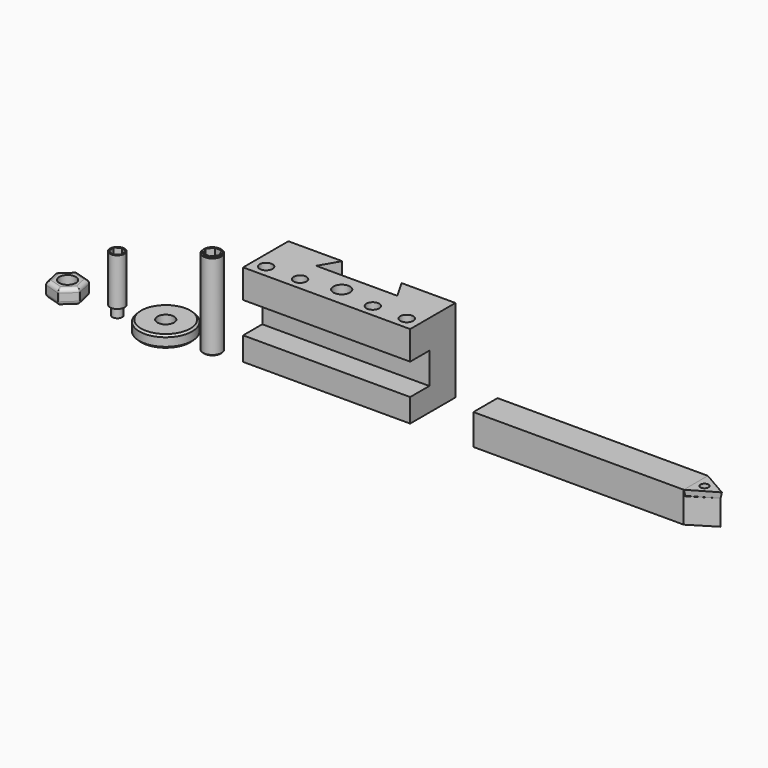
from build123d import *

# Parameters (mm, degrees)
F0_W      = 88.56
F0_H      = 12.4
F0_H_2    = 16.5
F0_H_3    = 15.22
F1_DEPTH  = 30
F2_DEPTH  = 12.7
F4_DEPTH  = 44.12
F5_D      = 6.8
F5_DEPTH  = 15.75
F5_TIP    = 2.0429261047
F6_D      = 8.8
F6_DEPTH  = 12
F6_TIP    = 2.6437867237
F7_R      = 4.9
F8_DEPTH  = 46
F9_SIZE   = 0.5
F11_DEPTH = 5
F12_R     = 14
F13_DEPTH = 6.43
F14_SIZE  = 1
F15_D     = 8.8
F16_R     = 2.6
F17_DEPTH = 5
F18_R     = 3.85
F19_DEPTH = 25
F21_DEPTH = 6.4
F23_DEPTH = 8
F24_D     = 8.8
F25_R     = 2
F26_R     = 0.5
F28_DEPTH = 16
F30_DEPTH = 13.3073726019
F32_DEPTH = 3
F32_TAPER = 7
F33_D     = 4.2
F33_DEPTH = 3
F33_TIP   = 1.2618073
F35_D     = 3.3


# Not quite as in the source:
# - a feature of the source that left no trace in its solid (it failed there, or was rolled back) is left out


with BuildPart() as f1:
    # F0 (on Front) → F1 (new body)
    with BuildSketch(Plane.XZ):
        with Locations((44.28, 6.2)):
            Rectangle(F0_W, F0_H)
        with Locations((44.28, 20.65)):
            Rectangle(F0_W, F0_H_2)
        with Locations((44.28, 36.51)):
            Rectangle(F0_W, F0_H_3)
    extrude(amount=-F1_DEPTH)

    # F0 (on Front) → F2 (cut)
    with BuildSketch(Plane.XZ):
        with Locations((44.28, 20.65)):
            Rectangle(F0_W, F0_H_2)
    extrude(amount=-F2_DEPTH, mode=Mode.SUBTRACT)

    # F3 (on face) → F4 (cut, through all)
    with BuildSketch(Plane.XY.offset(44.12)):
        Polygon((28.5535026919, 30), (22.78, 20), (65.78, 20), (60.0064973081, 30), align=None)
    extrude(amount=-F4_DEPTH, mode=Mode.SUBTRACT)

    # F5
    with Locations(Plane.XY.offset(44.12)):
        with Locations((7, 6.5), (25, 6.5), (63.56, 6.5), (81.56, 6.5)):
            Hole(F5_D / 2, depth=F5_DEPTH)
            with Locations((0, 0, -(F5_DEPTH + F5_TIP / 2))):  # 118° drill point
                Cone(0, F5_D / 2, F5_TIP, mode=Mode.SUBTRACT)

    # F6
    with Locations(Plane.XY.offset(44.12)):
        with Locations((44.28, 10)):
            Hole(F6_D / 2, depth=F6_DEPTH)
            with Locations((0, 0, -(F6_DEPTH + F6_TIP / 2))):  # 118° drill point
                Cone(0, F6_D / 2, F6_TIP, mode=Mode.SUBTRACT)


with BuildPart() as f8:
    # F7 (on Top) → F8 (new body)
    with BuildSketch(Plane.XY):
        with Locations((-16.2864004874, 0)):
            Circle(F7_R)
    extrude(amount=F8_DEPTH)

    # F9
    f9_edges = [f8.edges().sort_by_distance(p)[0] for p in [
        (-21.1864, 0, 46),
        (-21.1864, 0, 0),
    ]]
    chamfer(f9_edges, length=F9_SIZE)

    # F10 (on face) → F11 (cut)
    with BuildSketch(Plane.XY.offset(46)):
        Polygon((-12.317548746, -0.4982126603), (-13.8705097964, 3.1880201018), (-17.8393615378, 3.686232762), (-20.2552522288, 0.4982126603), (-18.7022911783, -3.1880201018), (-14.733439437, -3.686232762), align=None)
    extrude(amount=-F11_DEPTH, mode=Mode.SUBTRACT)


with BuildPart() as f13:
    # F12 (on Top) → F13 (new body)
    with BuildSketch(Plane.XY):
        with Locations((-41.0129390657, 0)):
            Circle(F12_R)
    extrude(amount=F13_DEPTH)

    # F14
    f14_edges = [f13.edges().sort_by_distance(p)[0] for p in [
        (-55.012939, 0, 6.43),
        (-55.012939, 0, 0),
    ]]
    chamfer(f14_edges, length=F14_SIZE)

    # F15 (through all)
    with Locations(Plane(origin=(0, 0, 0), x_dir=(1, 0, 0), z_dir=(0, 0, -1))):
        with Locations((-41.0129390657, 0)):
            Hole(F15_D / 2)


with BuildPart() as f17:
    # F16 (on Top) → F17 (new body)
    with BuildSketch(Plane.XY):
        with Locations((-66.6916072369, 0)):
            Circle(F16_R)
    extrude(amount=F17_DEPTH)

    # F18 (on face) → F19 (join)
    with BuildSketch(Plane.XY.offset(5)):
        with Locations((-66.6916072369, 0)):
            Circle(F18_R)
    extrude(amount=F19_DEPTH)

    # F20 (on face) → F21 (cut)
    with BuildSketch(Plane.XY.offset(30)):
        Polygon((-63.8243739041, 2.007230185), (-66.9963029019, 3.4867119972), (-69.8635362347, 1.4794818123), (-69.5588405696, -2.007230185), (-66.3869115718, -3.4867119972), (-63.519678239, -1.4794818123), align=None)
    extrude(amount=-F21_DEPTH, mode=Mode.SUBTRACT)


with BuildPart() as f23:
    # F22 (on Top) → F23 (new body)
    with BuildSketch(Plane.XY):
        Polygon((-84.449759066, -2.6274492815), (-86.4782877336, 6.1409639983), (-95.0862207185, 8.7684132798), (-101.6656250359, 2.6274492815), (-99.6370963683, -6.1409639983), (-91.0291633834, -8.7684132798), align=None)
    extrude(amount=F23_DEPTH)

    # F24 (through all)
    with Locations(Plane(origin=(0, 0, 0), x_dir=(1, 0, 0), z_dir=(0, 0, -1))):
        with Locations((-93.0576920509, 0)):
            Hole(F24_D / 2)

    # F25
    f25_edges = [f23.edges().sort_by_distance(p)[0] for p in [
        (-98.375923, 5.697931, 8),
        (-90.782254, 7.454689, 8),
        (-85.464023, 1.756757, 8),
        (-87.739461, -5.697931, 8),
        (-95.33313, -7.454689, 8),
        (-100.651361, -1.756757, 8),
        (-100.651361, -1.756757, 0),
        (-98.375923, 5.697931, 0),
        (-90.782254, 7.454689, 0),
        (-85.464023, 1.756757, 0),
        (-87.739461, -5.697931, 0),
        (-95.33313, -7.454689, 0),
    ]]
    fillet(f25_edges, radius=F25_R)

    # F26
    f26_edges = [f23.edges().sort_by_distance(p)[0] for p in [
        (-99.637096, -6.140964, 4),
        (-91.029163, -8.768413, 4),
        (-84.449759, -2.627449, 4),
        (-101.665625, 2.627449, 4),
        (-95.086221, 8.768413, 4),
        (-86.478288, 6.140964, 4),
        (-91.18162, -8.109411, 0.585786),
        (-85.096701, -2.42998, 0.585786),
        (-91.18162, -8.109411, 7.414214),
        (-85.096701, -2.42998, 7.414214),
        (-99.142612, -5.679431, 0.585786),
        (-99.142612, -5.679431, 7.414214),
        (-86.972772, 5.679431, 0.585786),
        (-86.972772, 5.679431, 7.414214),
        (-101.018683, 2.42998, 0.585786),
        (-101.018683, 2.42998, 7.414214),
        (-94.933764, 8.109411, 0.585786),
        (-94.933764, 8.109411, 7.414214),
    ]]
    fillet(f26_edges, radius=F26_R)


with BuildPart() as f28:
    # F27 (on Front) → F28 (new body)
    with BuildSketch(Plane.XZ):
        Polygon((122.0868207611, 16.3073726019), (122.0868207611, 0), (245.4528808594, 0), (246.5868207611, 0), (246.5868207611, 13.3073726019), (233.5868207611, 13.3073726019), (233.5868207611, 16.3073726019), align=None)
    extrude(amount=-F28_DEPTH)

    # F29 (on face) → F30 (cut, through all)
    with BuildSketch(Plane.XY.offset(13.3073726019)):
        Polygon((246.5868207611, 16), (233.5868207611, 16), (246.5868207611, 8), align=None)
        Polygon((246.5868207611, 0), (246.5868207611, 8), (233.5868207611, 0), align=None)
    extrude(amount=-F30_DEPTH, mode=Mode.SUBTRACT)

    # F35 (through all)
    with Locations(Plane(origin=(0, 0, 0), x_dir=(1, 0, 0), z_dir=(0, 0, -1))):
        with Locations((238.2056229146, -8)):
            Hole(F35_D / 2)


with BuildPart() as f32:
    # F31 (on face) → F32 (new body)
    with BuildSketch(Plane.XY.offset(16.3073726019)):
        Polygon((233.5868207611, 16), (233.5868207611, 0), (247.4432272216, 8), align=None)
    extrude(amount=-F32_DEPTH, taper=F32_TAPER)

    # F33
    with Locations(Plane.XY.offset(16.3073726019)):
        with Locations((238.2056229146, 8)):
            Hole(F33_D / 2, depth=F33_DEPTH)
            with Locations((0, 0, -(F33_DEPTH + F33_TIP / 2))):  # 118° drill point
                Cone(0, F33_D / 2, F33_TIP, mode=Mode.SUBTRACT)


solid = Compound([f1.part, f8.part, f13.part, f17.part, f23.part, f28.part, f32.part])
